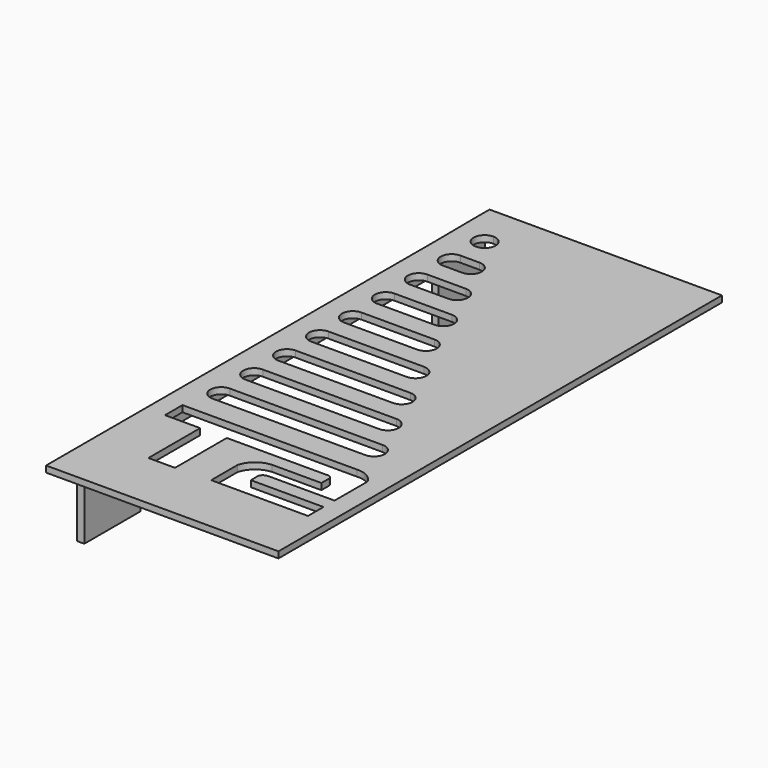
from build123d import *

# Parameters (mm, degrees)
F1_DEPTH = 1.3
F2_DEPTH = 17
F4_DEPTH = 5


# Not quite as in the source:
# - a feature names something its author has since deleted; it is built from what else it names


with BuildPart() as f1:
    # F0 (on Top) → F1 (new body)
    with BuildSketch(Plane.XY):
        Polygon((24, 57.25), (-24, 57.25), (-24.0091441598, 54.25), (-22.5091511277, 54.2454279414), (-22.5091511277, 42.2454279414), (-22.4957785658, -34.7500035641), (-22.5, -49.25), (-24, -49.25), (-24, -57.25), (24, -57.25), align=None)
        with BuildLine():
            Line((13.9209458456, -22.2416133583), (-17.6390541544, -22.2416133583))
            ThreePointArc((-17.6390541544, -22.2416133583), (-19.8890541544, -19.9916133583), (-17.6390541544, -17.7416133583))
            Line((-17.6390541544, -17.7416133583), (13.9209458456, -17.7416133583))
            ThreePointArc((13.9209458456, -17.7416133583), (16.1709458456, -19.9916133583), (13.9209458456, -22.2416133583))
        make_face(mode=Mode.SUBTRACT)
        with BuildLine():
            Line((9.9809458456, -13.7416133583), (-17.6390541544, -13.7416133583))
            ThreePointArc((-17.6390541544, -13.7416133583), (-19.8890541544, -11.4916133583), (-17.6390541544, -9.2416133583))
            Line((-17.6390541544, -9.2416133583), (9.9809458456, -9.2416133583))
            ThreePointArc((9.9809458456, -9.2416133583), (12.2309458456, -11.4916133583), (9.9809458456, -13.7416133583))
        make_face(mode=Mode.SUBTRACT)
        with BuildLine():
            Line((6.0409458456, -5.2416133583), (-17.6390541544, -5.2416133583))
            ThreePointArc((-17.6390541544, -5.2416133583), (-19.8890541544, -2.9916133583), (-17.6390541544, -0.7416133583))
            Line((-17.6390541544, -0.7416133583), (6.0409458456, -0.7416133583))
            ThreePointArc((6.0409458456, -0.7416133583), (8.2909458456, -2.9916133583), (6.0409458456, -5.2416133583))
        make_face(mode=Mode.SUBTRACT)
        with BuildLine():
            Line((-19.9999999992, -31.5317022603), (-19.9999999992, -27.0317022603))
            Line((-19.9999999992, -27.0317022603), (16.0951670268, -27.0317022603))
            ThreePointArc((16.0951670268, -27.0317022603), (18.3824934665, -27.555243649), (19.9999999704, -29.25513498))
            Line((19.9999999704, -29.25513498), (19.991580365, -37.75513498))
            Line((19.991580365, -37.75513498), (6.1573753969, -37.7551350426))
            ThreePointArc((6.1573753969, -37.7551350426), (5.4441089744, -38.037790108), (4.9890264818, -38.6554816172))
            Line((4.9890264818, -38.6554816172), (4.9890264818, -40.6197120801))
            Line((4.9890264818, -40.6197120801), (19.9890264818, -40.6197120801))
            Line((19.9890264818, -40.6197120801), (20, -44.6197120801))
            Line((20, -44.6197120801), (0, -44.6197120801))
            Line((0, -44.6197120801), (0, -37.7900532508))
            ThreePointArc((0, -37.7900532508), (1.5958871284, -35.3350022858), (4.3312619815, -34.2900834468))
            Line((4.3312619815, -34.2900834468), (14.5000001306, -34.2900834468))
            Line((14.5000001306, -34.2900834468), (14.5000000048, -32.3122422563))
            ThreePointArc((14.5000000048, -32.3122422563), (14.2713851276, -31.7603171319), (13.7194600008, -31.5317022603))
            Line((13.7194600008, -31.5317022603), (-7.2499999992, -31.5317022603))
            Line((-7.2499999992, -31.5317022603), (-7.2499999992, -44.8960133593))
            Line((-7.2499999992, -44.8960133593), (-12.7499999992, -44.8960133593))
            Line((-12.7499999992, -44.8960133593), (-12.7499999992, -31.5317022603))
            Line((-12.7499999992, -31.5317022603), (-19.9999999992, -31.5317022603))
        make_face(mode=Mode.SUBTRACT)
        with BuildLine():
            Line((2.1009458456, 3.2583866417), (-17.6390541544, 3.2583866417))
            ThreePointArc((-17.6390541544, 3.2583866417), (-19.8890541544, 5.5083866417), (-17.6390541544, 7.7583866417))
            Line((-17.6390541544, 7.7583866417), (2.1009458456, 7.7583866417))
            ThreePointArc((2.1009458456, 7.7583866417), (4.3509458456, 5.5083866417), (2.1009458456, 3.2583866417))
        make_face(mode=Mode.SUBTRACT)
        with BuildLine():
            Line((-2.5590541544, 11.7583866417), (-17.6390541544, 11.7583866417))
            ThreePointArc((-17.6390541544, 11.7583866417), (-19.8890541544, 14.0083866417), (-17.6390541544, 16.2583866417))
            Line((-17.6390541544, 16.2583866417), (-2.5590541544, 16.2583866417))
            ThreePointArc((-2.5590541544, 16.2583866417), (-0.3090541544, 14.0083866417), (-2.5590541544, 11.7583866417))
        make_face(mode=Mode.SUBTRACT)
        with BuildLine():
            Line((-5.7790541544, 20.2583866417), (-17.6390541544, 20.2583866417))
            ThreePointArc((-17.6390541544, 20.2583866417), (-19.8890541544, 22.5083866417), (-17.6390541544, 24.7583866417))
            Line((-17.6390541544, 24.7583866417), (-5.7790541544, 24.7583866417))
            ThreePointArc((-5.7790541544, 24.7583866417), (-3.5290541544, 22.5083866417), (-5.7790541544, 20.2583866417))
        make_face(mode=Mode.SUBTRACT)
        with BuildLine():
            Line((-9.7190541544, 28.7583866417), (-17.6390541544, 28.7583866417))
            ThreePointArc((-17.6390541544, 28.7583866417), (-19.8890541544, 31.0083866417), (-17.6390541544, 33.2583866417))
            Line((-17.6390541544, 33.2583866417), (-9.7190541544, 33.2583866417))
            ThreePointArc((-9.7190541544, 33.2583866417), (-7.4690541544, 31.0083866417), (-9.7190541544, 28.7583866417))
        make_face(mode=Mode.SUBTRACT)
        with BuildLine():
            Line((-13.6590541544, 37.2583866417), (-17.6390541544, 37.2583866417))
            ThreePointArc((-17.6390541544, 37.2583866417), (-19.8890541544, 39.5083866417), (-17.6390541544, 41.7583866417))
            Line((-17.6390541544, 41.7583866417), (-13.6590541544, 41.7583866417))
            ThreePointArc((-13.6590541544, 41.7583866417), (-11.4090541544, 39.5083866417), (-13.6590541544, 37.2583866417))
        make_face(mode=Mode.SUBTRACT)
        with BuildLine():
            Line((-17.5990541544, 45.7583866417), (-17.6390541544, 45.7583866417))
            ThreePointArc((-17.6390541544, 45.7583866417), (-19.8890541544, 48.0083866417), (-17.6390541544, 50.2583866417))
            Line((-17.6390541544, 50.2583866417), (-17.5990541544, 50.2583866417))
            ThreePointArc((-17.5990541544, 50.2583866417), (-15.3490541544, 48.0083866417), (-17.5990541544, 45.7583866417))
        make_face(mode=Mode.SUBTRACT)
    extrude(amount=-F1_DEPTH)

    # F0 (on Top) → F2 (join)
    with BuildSketch(Plane.XY):
        Polygon((-22.5091511277, 54.2454279414), (-24.0091441598, 54.25), (-23.9065294749, 42.2334950591), (-22.5091511277, 42.2454279414), align=None)
        Polygon((-22.4957785658, -34.7500035641), (-23.9957785658, -34.7500035641), (-24, -49.25), (-22.5, -49.25), align=None)
    extrude(amount=-F2_DEPTH)

    # F0 (on Top) → F4 (join)
    with BuildSketch(Plane.XY):
        Polygon((-22.5091511277, 42.2454279414), (-23.9065294749, 42.2334950591), (-23.9957785658, -34.7500035641), (-22.4957785658, -34.7500035641), align=None)
    extrude(amount=-F4_DEPTH)


solid = f1.part
